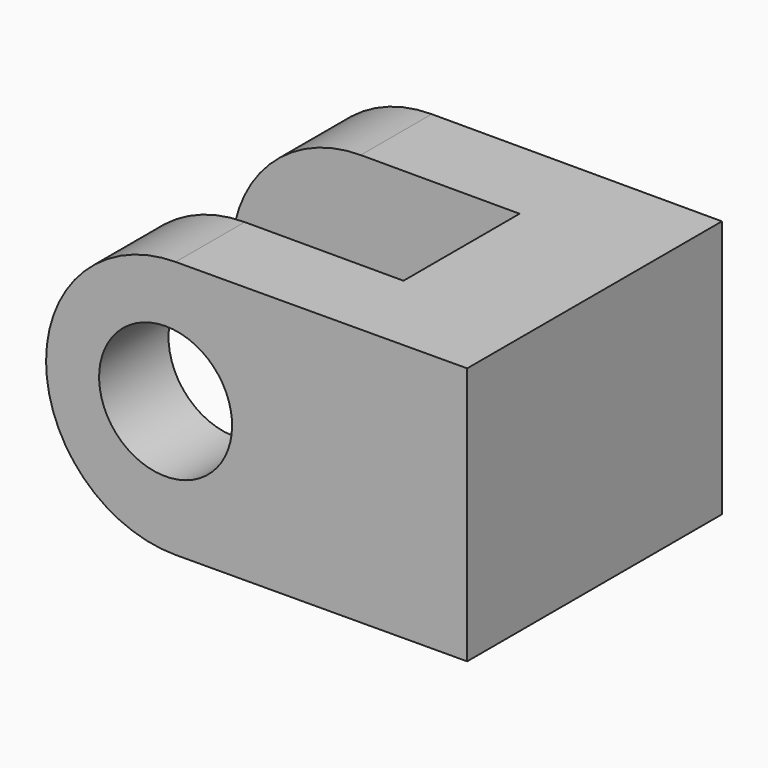
from build123d import *

# Parameters (mm, degrees)
F1_DEPTH = 32
F2_R     = 16
F3_R     = 16
F4_R     = 15.99999
F5_R     = 15.99999
F6_R     = 8.20953723
F7_DEPTH = 16


# Not quite as in the source:
# - a fillet or chamfer is up to 0.001 mm smaller than in the source, because OpenCascade refuses the exact size


with BuildPart() as f1:
    # F0 (on Top) → F1 (new body)
    with BuildSketch(Plane.XY):
        Polygon((43.1044374643, -14.2427797436), (43.1044374643, 25.2572197622), (-8.8955625357, 25.2572197622), (-8.8955625357, 14.2572197622), (26.8044351456, 14.2572197622), (26.8044351456, -3.7427802378), (-8.8955625357, -3.7427802378), (-8.8955625357, -14.5427802378), align=None)
    extrude(amount=F1_DEPTH)

    # F2
    f2_edges = [f1.edges().sort_by_distance(p)[0] for p in [
        (-8.895563, -9.14278, 32),
    ]]
    fillet(f2_edges, radius=F2_R)

    # F3
    f3_edges = [f1.edges().sort_by_distance(p)[0] for p in [
        (-8.895563, 19.75722, 32),
    ]]
    fillet(f3_edges, radius=F3_R)

    # F4 (radius 16 in the source; OpenCascade refuses exactly that, so slightly less here)
    f4_edges = [f1.edges().sort_by_distance(p)[0] for p in [
        (-8.895563, 19.75722, 0),
    ]]
    fillet(f4_edges, radius=F4_R)

    # F5 (radius 16 in the source; OpenCascade refuses exactly that, so slightly less here)
    f5_edges = [f1.edges().sort_by_distance(p)[0] for p in [
        (-8.895563, -9.14278, 0),
    ]]
    fillet(f5_edges, radius=F5_R)

    # F6 (on Front) → F7 (cut)
    with BuildSketch(Plane.XZ):
        with Locations((5.8611659333, 16.3812022656)):
            Circle(F6_R)
    extrude(amount=F7_DEPTH, mode=Mode.SUBTRACT)


solid = f1.part
